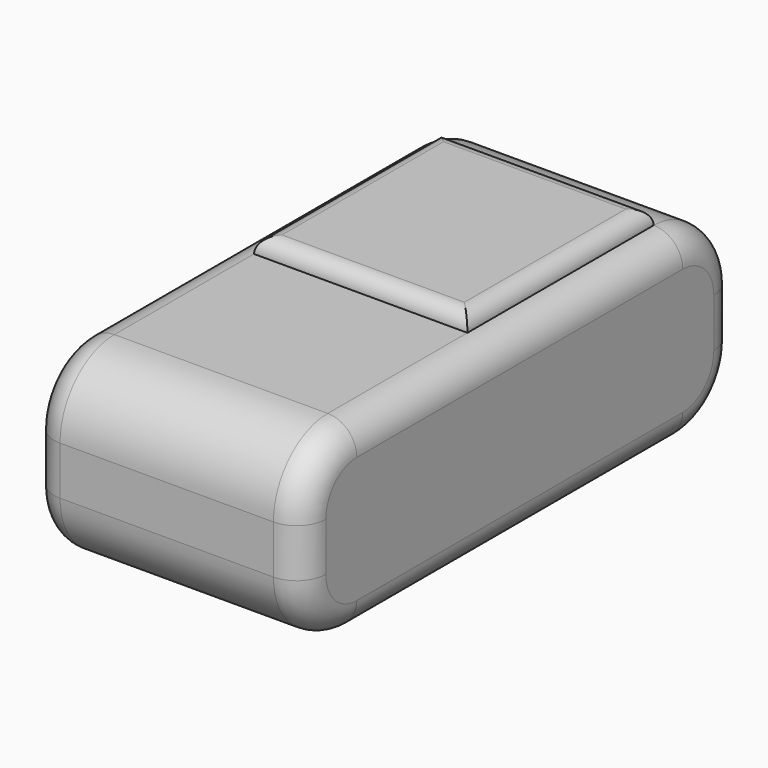
from build123d import *

# Parameters (mm, degrees)
F0_W         = 140
F0_H         = 280
F1_DEPTH     = 95
F2_R         = 15
F3_T1_DEPTH  = 140
F3_T4_ANGLE  = 90
F3_T6_ANGLE  = 90
F3_T8_ANGLE  = 90
F3_T10_ANGLE = 90
F3_T12_ANGLE = 90
F3_T14_ANGLE = 90
F3_T16_ANGLE = 90
F3_T18_ANGLE = 90
F4_W         = 110
F4_H         = 120
F5_DEPTH     = 8
F6_R         = 7.99999


# Not quite as in the source:
# - a fillet or chamfer that OpenCascade refuses, or shapes differently, is made with other operations: its cross-section is extruded or revolved along the edge and cut away or added
# - a fillet or chamfer is up to 0.001 mm smaller than in the source, because OpenCascade refuses the exact size


with BuildPart() as f1:
    # F0 (on Top) → F1 (new body)
    with BuildSketch(Plane.XY):
        Rectangle(F0_W, F0_H)
    extrude(amount=F1_DEPTH)

    # F2
    f2_edges = [f1.edges().sort_by_distance(p)[0] for p in [
        (70, -140, 47.5),
        (70, 140, 47.5),
        (70, 0, 0),
        (70, 0, 95),
        (-70, 140, 47.5),
        (-70, -140, 47.5),
        (-70, 0, 0),
        (-70, 0, 95),
    ]]
    fillet(f2_edges, radius=F2_R)

    # F3: fillet of radius 35 on 4 edges, made by hand

    # F3_s2 → F3_t1 (cut)
    with BuildSketch(Plane.YZ.offset(-70)):
        with BuildLine():
            ThreePointArc((-140, 60), (-129.7487373415, 84.7487373415), (-105, 95))
            Line((-105, 95), (-140, 95))
            Line((-140, 95), (-140, 60))
        make_face()
        with BuildLine():
            ThreePointArc((-140, 35), (-129.7487373415, 10.2512626585), (-105, 0))
            Line((-105, 0), (-140, 0))
            Line((-140, 0), (-140, 35))
        make_face()
        with BuildLine():
            ThreePointArc((105, 95), (129.7487373415, 84.7487373415), (140, 60))
            Line((140, 60), (140, 95))
            Line((140, 95), (105, 95))
        make_face()
        with BuildLine():
            ThreePointArc((105, 0), (129.7487373415, 10.2512626585), (140, 35))
            Line((140, 35), (140, 0))
            Line((140, 0), (105, 0))
        make_face()
    extrude(amount=F3_T1_DEPTH, mode=Mode.SUBTRACT)

    # F3_s3 → F3_t4 (revolve, cut)
    with BuildSketch(Plane.XZ.offset(-105)):
        with BuildLine():
            ThreePointArc((70, 15), (65.6066017178, 4.3933982822), (55, 0))
            Line((55, 0), (70, 0))
            Line((70, 0), (70, 15))
        make_face()
    revolve(axis=Axis((70, 105, 35), (1, 0, 0)), revolution_arc=F3_T4_ANGLE, mode=Mode.SUBTRACT)

    # F3_s5 → F3_t6 (revolve, cut)
    with BuildSketch(Plane.XY.offset(35)):
        with BuildLine():
            ThreePointArc((-70, 125), (-65.6066017178, 135.6066017178), (-55, 140))
            Line((-55, 140), (-70, 140))
            Line((-70, 140), (-70, 125))
        make_face()
    revolve(axis=Axis((-70, 105, 35), (-1, 0, 0)), revolution_arc=F3_T6_ANGLE, mode=Mode.SUBTRACT)

    # F3_s7 → F3_t8 (revolve, cut)
    with BuildSketch(Plane.XY.offset(60)):
        with BuildLine():
            ThreePointArc((70, 125), (65.6066017178, 135.6066017178), (55, 140))
            Line((55, 140), (70, 140))
            Line((70, 140), (70, 125))
        make_face()
    revolve(axis=Axis((70, 105, 60), (1, 0, 0)), revolution_arc=F3_T8_ANGLE, mode=Mode.SUBTRACT)

    # F3_s9 → F3_t10 (revolve, cut)
    with BuildSketch(Plane.XZ.offset(-105)):
        with BuildLine():
            ThreePointArc((-70, 80), (-65.6066017178, 90.6066017178), (-55, 95))
            Line((-55, 95), (-70, 95))
            Line((-70, 95), (-70, 80))
        make_face()
    revolve(axis=Axis((-70, 105, 60), (-1, 0, 0)), revolution_arc=F3_T10_ANGLE, mode=Mode.SUBTRACT)

    # F3_s11 → F3_t12 (revolve, cut)
    with BuildSketch(Plane.XZ.offset(105)):
        with BuildLine():
            ThreePointArc((-70, 15), (-65.6066017178, 4.3933982822), (-55, 0))
            Line((-55, 0), (-70, 0))
            Line((-70, 0), (-70, 15))
        make_face()
    revolve(axis=Axis((-70, -105, 35), (-1, 0, 0)), revolution_arc=F3_T12_ANGLE, mode=Mode.SUBTRACT)

    # F3_s13 → F3_t14 (revolve, cut)
    with BuildSketch(Plane.XY.offset(35)):
        with BuildLine():
            ThreePointArc((70, -125), (65.6066017178, -135.6066017178), (55, -140))
            Line((55, -140), (70, -140))
            Line((70, -140), (70, -125))
        make_face()
    revolve(axis=Axis((70, -105, 35), (1, 0, 0)), revolution_arc=F3_T14_ANGLE, mode=Mode.SUBTRACT)

    # F3_s15 → F3_t16 (revolve, cut)
    with BuildSketch(Plane.XY.offset(60)):
        with BuildLine():
            ThreePointArc((-70, -125), (-65.6066017178, -135.6066017178), (-55, -140))
            Line((-55, -140), (-70, -140))
            Line((-70, -140), (-70, -125))
        make_face()
    revolve(axis=Axis((-70, -105, 60), (-1, 0, 0)), revolution_arc=F3_T16_ANGLE, mode=Mode.SUBTRACT)

    # F3_s17 → F3_t18 (revolve, cut)
    with BuildSketch(Plane.XZ.offset(105)):
        with BuildLine():
            ThreePointArc((70, 80), (65.6066017178, 90.6066017178), (55, 95))
            Line((55, 95), (70, 95))
            Line((70, 95), (70, 80))
        make_face()
    revolve(axis=Axis((70, -105, 60), (1, 0, 0)), revolution_arc=F3_T18_ANGLE, mode=Mode.SUBTRACT)

    # F4 (on face) → F5 (join)
    with BuildSketch(Plane.XY.offset(95)):
        with Locations((0, 45)):
            Rectangle(F4_W, F4_H)
    extrude(amount=F5_DEPTH)

    # F6 (radius 8 in the source; OpenCascade refuses exactly that, so slightly less here)
    f6_edges = [f1.edges().sort_by_distance(p)[0] for p in [
        (0, 105, 103),
        (-55, 45, 103),
        (0, -15, 103),
        (55, 45, 103),
    ]]
    fillet(f6_edges, radius=F6_R)


solid = f1.part
